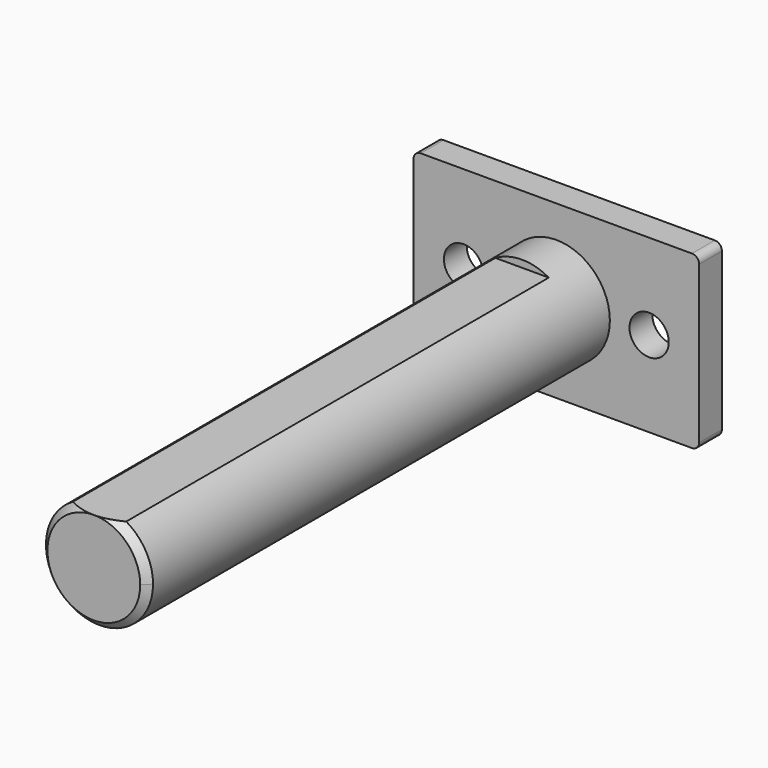
from build123d import *

# Parameters (mm, degrees)
F0_W        = 40
F0_H        = 24
F0_R        = 2.5
F0_R_2      = 7.5
F1_DEPTH    = 4
F3_DEPTH    = 81
F4_D        = 5.5
F4_DEPTH    = 4
F4_TIP      = 1.6523667023
F6_DEPTH    = 75
F7_T2_ANGLE = 287.359476763
F7_T4_ANGLE = 107.2329087186
F8_R        = 7.5
F9_DEPTH    = 2
F10_R       = 1


# Not quite as in the source:
# - a fillet or chamfer that OpenCascade refuses, or shapes differently, is made with other operations: its cross-section is extruded or revolved along the edge and cut away or added


with BuildPart() as f1:
    # F0 (on Front) → F1 (new body)
    with BuildSketch(Plane.XZ):
        with Locations((20, 12)):
            Rectangle(F0_W, F0_H)
        with Locations((7, 12)):
            Circle(F0_R, mode=Mode.SUBTRACT)
        with Locations((20, 12)):
            Circle(F0_R_2, mode=Mode.SUBTRACT)
        with Locations((33, 12)):
            Circle(F0_R, mode=Mode.SUBTRACT)
        with Locations((20, 12)):
            Circle(F0_R_2)
        with Locations((7, 12)):
            Circle(F0_R)
        with Locations((33, 12)):
            Circle(F0_R)
    extrude(amount=-F1_DEPTH)

    # F0 (on Front) → F3 (join)
    with BuildSketch(Plane.XZ):
        with Locations((20, 12)):
            Circle(F0_R_2)
    extrude(amount=F3_DEPTH)

    # F4
    with Locations(Plane.XZ):
        with Locations((33, 12), (7, 12)):
            Hole(F4_D / 2, depth=F4_DEPTH)
            with Locations((0, 0, -(F4_DEPTH + F4_TIP / 2))):  # 118° drill point
                Cone(0, F4_D / 2, F4_TIP, mode=Mode.SUBTRACT)

    # F5 (on face) → F6 (cut)
    with BuildSketch(Plane.XZ.offset(81)):
        with BuildLine():
            ThreePointArc((23.7416573868, 18.5), (20, 19.5), (16.2583426132, 18.5))
            Line((16.2583426132, 18.5), (23.7416573868, 18.5))
        make_face()
    extrude(amount=-F6_DEPTH, mode=Mode.SUBTRACT)

    # F7: chamfer of 1 on 2 edges, made by hand

    # F7_s1 → F7_t2 (revolve, cut)
    with BuildSketch(Plane(origin=(14.8022480235, 0, -4.6272486525), x_dir=(0, 1, 0), z_dir=(0.9544515906, 0, -0.2983658178))):
        with BuildLine():
            Line((-79.9717157288, 24.9490197138), (-81.0282842712, 23.8924511713))
            Line((-81.0282842712, 23.8924511713), (-81.0482842712, 23.8924511713))
            ThreePointArc((-81.0482842712, 23.8924511713), (-81.02, 24.406593307), (-81.02, 24.9207354426))
            Line((-81.02, 24.9207354426), (-81, 24.9407354426))
            ThreePointArc((-81, 24.9407354426), (-80.4858578644, 24.9407354426), (-79.9717157288, 24.9690197138))
            Line((-79.9717157288, 24.9690197138), (-79.9717157288, 24.9490197138))
        make_face()
    revolve(axis=Axis((20, -81, 12), (0, -1, 0)), revolution_arc=F7_T2_ANGLE, mode=Mode.SUBTRACT)

    # F7_s3 → F7_t4 (revolve, cut)
    with BuildSketch(Plane.XY.offset(12)):
        with BuildLine():
            Line((27.5282842712, -79.9717157288), (26.4717157288, -81.0282842712))
            Line((26.4717157288, -81.0282842712), (26.4717157288, -81.0482842712))
            ThreePointArc((26.4717157288, -81.0482842712), (26.9858578644, -81.02), (27.5, -81.02))
            Line((27.5, -81.02), (27.52, -81))
            ThreePointArc((27.52, -81), (27.52, -80.4858578644), (27.5482842712, -79.9717157288))
            Line((27.5482842712, -79.9717157288), (27.5282842712, -79.9717157288))
        make_face()
    revolve(axis=Axis((20, -81, 12), (0, -1, 0)), revolution_arc=F7_T4_ANGLE, mode=Mode.SUBTRACT)

    # F8 (on face) → F9 (cut)
    with BuildSketch(Plane(origin=(0, 4, 0), x_dir=(-1, 0, 0), z_dir=(0, 1, 0))):
        with Locations((-20, 12)):
            Circle(F8_R)
    extrude(amount=-F9_DEPTH, mode=Mode.SUBTRACT)

    # F10
    f10_edges = [f1.edges().sort_by_distance(p)[0] for p in [
        (0, 2, 24),
        (0, 2, 0),
        (40, 2, 0),
        (40, 2, 24),
        (27.5, 2, 12),
    ]]
    fillet(f10_edges, radius=F10_R)


solid = f1.part
